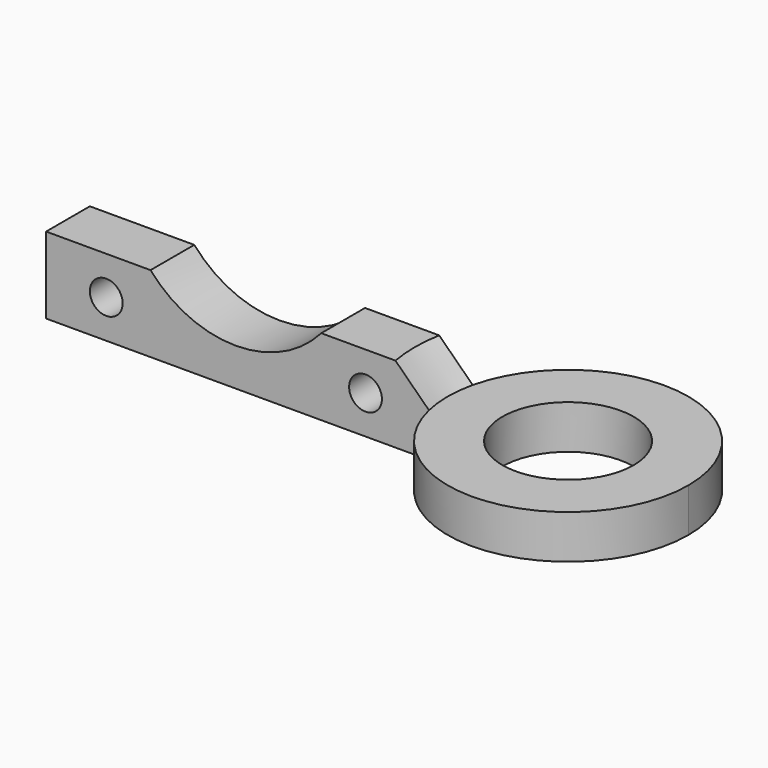
from build123d import *

# Parameters (mm, degrees)
F0_R     = 6
F1_DEPTH = 4
F0_W     = 1.5
F0_H     = 5
F0_W_2   = 10.35
F0_W_3   = 4
F2_DEPTH = 7
F6_SIZE  = 2.99999


# Not quite as in the source:
# - a fillet or chamfer is up to 0.001 mm smaller than in the source, because OpenCascade refuses the exact size


with BuildPart() as f1:
    # F0 (on Top) → F1 (new body)
    with BuildSketch(Plane.XY):
        with BuildLine():
            ThreePointArc((-10.7121426428, -2.5), (1.258258902, -10.9277987049), (11, 0))
            ThreePointArc((11, 0), (1.258258902, 10.9277987049), (-10.7121426428, 2.5))
            ThreePointArc((-10.7121426428, 2.5), (-11, 0), (-10.7121426428, -2.5))
        make_face()
        Circle(F0_R, mode=Mode.SUBTRACT)
    extrude(amount=F1_DEPTH)

    # F0 (on Top) → F2 (join)
    with BuildSketch(Plane.XY):
        with BuildLine():
            ThreePointArc((-10.7121426428, -2.5), (-11, 0), (-10.7121426428, 2.5))
            Line((-10.7121426428, 2.5), (-15.0121426428, 2.5))
            Line((-15.0121426428, 2.5), (-15.0121426428, -2.5))
            Line((-15.0121426428, -2.5), (-10.7121426428, -2.5))
        make_face()
        with Locations((-15.7621426428, 0)):
            Rectangle(F0_W, F0_H)
        with Locations((-17.2621426428, 0)):
            Rectangle(F0_W, F0_H)
        with Locations((-33.5371426428, 0)):
            Rectangle(F0_W_2, F0_H)
        with Locations((-39.4621426428, 0)):
            Rectangle(F0_W, F0_H)
        with Locations((-40.9621426428, 0)):
            Rectangle(F0_W, F0_H)
        with Locations((-43.7121426428, 0)):
            Rectangle(F0_W_3, F0_H)
        with Locations((-23.1871426428, 0)):
            Rectangle(F0_W_2, F0_H)
    extrude(amount=F2_DEPTH)

    # F6 (size 3 in the source; OpenCascade refuses exactly that, so slightly less here)
    f6_edges = [f1.edges().sort_by_distance(p)[0] for p in [
        (-11, 0, 7),
    ]]
    chamfer(f6_edges, length=F6_SIZE)


with BuildPart() as f3:
    # F0 (on Top) → F3 (revolve)
    with BuildSketch(Plane.XY):
        with Locations((-15.7621426428, 0)):
            Rectangle(F0_W, F0_H)
    revolve(axis=Axis((-16.5121426428, 0, 0), (0, -1, 0)))


with BuildPart() as f4:
    # F0 (on Top) → F4 (revolve)
    with BuildSketch(Plane.XY):
        with Locations((-39.4621426428, 0)):
            Rectangle(F0_W, F0_H)
    revolve(axis=Axis((-40.2121426428, 0, 0), (0, -1, 0)))


with BuildPart() as f4_1:
    # F5: moved
    add(f4.part.moved(Location((0, 0, 3.5))))


with BuildPart() as f3_1:
    # F5: moved
    add(f3.part.moved(Location((0, 0, 3.5))))


with BuildPart() as f7:
    # F0 (on Top) → F7 (revolve)
    with BuildSketch(Plane.XY):
        with Locations((-23.1871426428, 0)):
            Rectangle(F0_W_2, F0_H)
    revolve(axis=Axis((-28.3621426428, 0, 0), (0, -1, 0)))


with BuildPart() as f7_1:
    # F8: moved
    add(f7.part.moved(Location((0, 0, 13.8))))


with BuildPart() as f1_1:
    add(f1.part)

    # F9: cut F4, F7, F3
    add(f4_1.part, mode=Mode.SUBTRACT)
    add(f7_1.part, mode=Mode.SUBTRACT)
    add(f3_1.part, mode=Mode.SUBTRACT)


solid = f1_1.part
